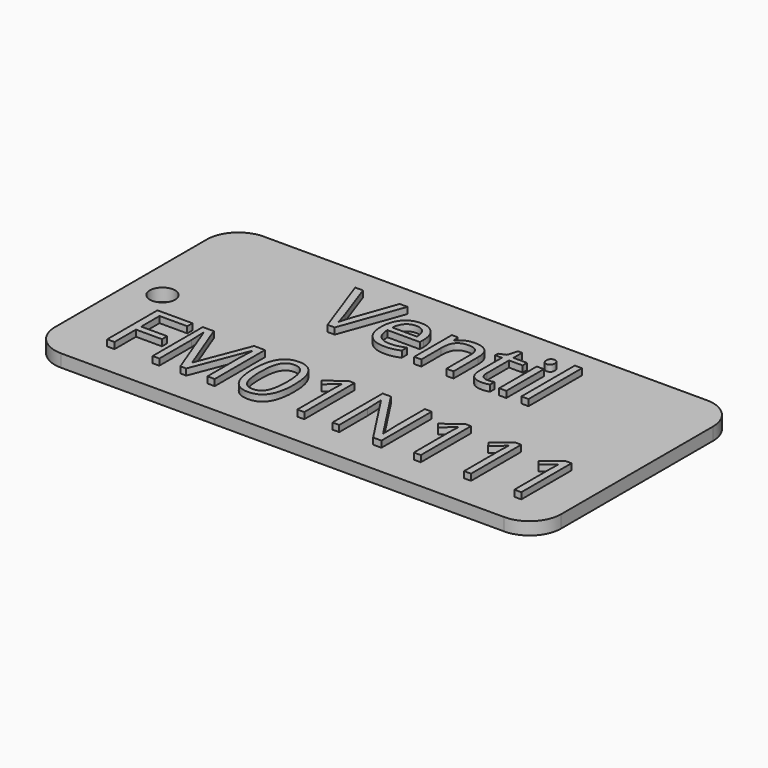
from build123d import *

# Parameters (mm, degrees)
F0_R         = 2
F1_DEPTH     = 2
F2_TEXT_SIZE = 13.8888888889
F3_DEPTH     = 1


# Not quite as in the source:
# - Text() gives the source's letters only with a copy of the font that has no kerning and outlines rounded to 1/6400 em; it was checked with that copy


with BuildPart() as f1:
    # F0 (on Top) → F1 (new body)
    with BuildSketch(Plane.XY):
        with BuildLine():
            Line((32.9065638036, 21.3038768982), (-37.0934361964, 21.3038768982))
            ThreePointArc((-37.0934361964, 21.3038768982), (-40.6289701024, 19.8394108041), (-42.0934361964, 16.3038768982))
            Line((-42.0934361964, 16.3038768982), (-42.0934361964, -13.6961231018))
            ThreePointArc((-42.0934361964, -13.6961231018), (-40.6289701024, -17.2316570078), (-37.0934361964, -18.6961231018))
            Line((-37.0934361964, -18.6961231018), (32.9065638036, -18.6961231018))
            ThreePointArc((32.9065638036, -18.6961231018), (36.4420977095, -17.2316570078), (37.9065638036, -13.6961231018))
            Line((37.9065638036, -13.6961231018), (37.9065638036, 16.3038768982))
            ThreePointArc((37.9065638036, 16.3038768982), (36.4420977095, 19.8394108041), (32.9065638036, 21.3038768982))
        make_face()
        with Locations((-37.0934361964, 1.3038768982)):
            Circle(F0_R, mode=Mode.SUBTRACT)
    extrude(amount=F1_DEPTH)

    # F2 (on face) → F3 (join)
    with BuildSketch(Plane.XY.offset(2)):
        with Locations((-18.574854359, 6.3038768982)):
            Text('Ventil', F2_TEXT_SIZE, font='Open Sans', text_align=(TextAlign.LEFT, TextAlign.BOTTOM))
        with Locations((-35.188253969, -13.6961231018)):
            Text('FM01N111', F2_TEXT_SIZE, font='Open Sans', text_align=(TextAlign.LEFT, TextAlign.BOTTOM))
    extrude(amount=F3_DEPTH)


solid = f1.part
